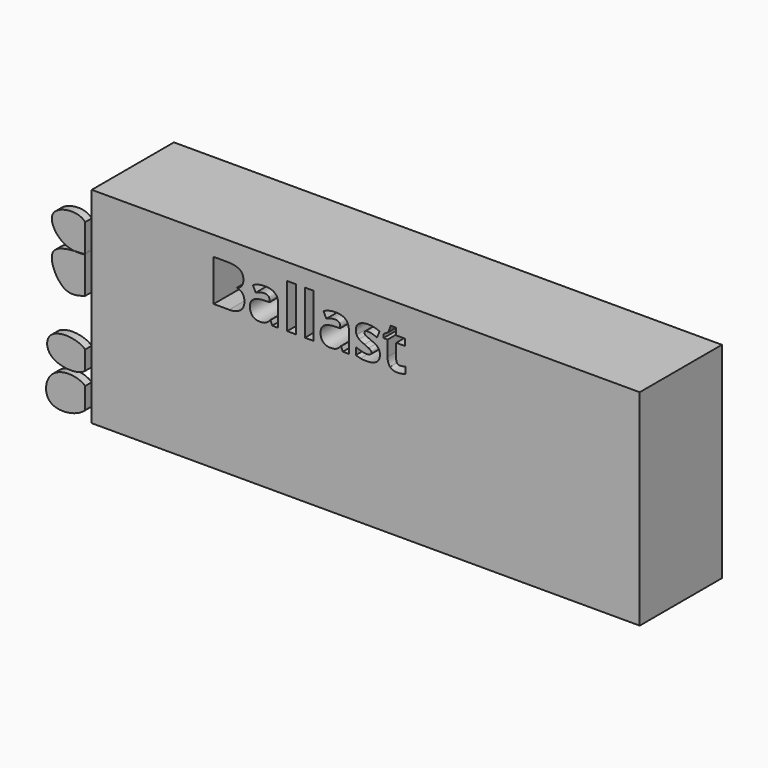
from build123d import *

# Parameters (mm, degrees)
F0_W     = 203.2
F0_H     = 76.2
F0_W_2   = 3.2102170287
F0_H_2   = 16.3812019001
F1_DEPTH = 38.1
F3_DEPTH = 3.048


with BuildPart() as f1:
    # F0 (on Front) → F1 (new body)
    with BuildSketch(Plane.XZ):
        with Locations((28.6630115066, 24.7132102959)):
            Rectangle(F0_W, F0_H)
        with BuildLine():
            Line((-27.7260044329, 40.2354274743), (-27.7260044329, 55.6262791053))
            Line((-27.7260044329, 55.6262791053), (-22.9359429272, 55.6262791053))
            add(Edge.make_bspline(
                [(-22.9359429272, 55.6262791053), (-19.6617236702, 55.6262791053), (-18.1829353432, 54.694878257)],
                knots=[0, 0, 0, 1, 1, 1], degree=2))
            add(Edge.make_bspline(
                [(-18.1829353432, 54.694878257), (-16.7041470162, 53.7634774087), (-16.7041470162, 51.7322487956)],
                knots=[0, 0, 0, 1, 1, 1], degree=2))
            add(Edge.make_bspline(
                [(-16.7041470162, 51.7322487956), (-16.7041470162, 50.3511480801), (-17.3509063756, 49.4669067684)],
                knots=[0, 0, 0, 1, 1, 1], degree=2))
            add(Edge.make_bspline(
                [(-17.3509063756, 49.4669067684), (-17.9976657351, 48.5826654567), (-19.0722294624, 48.4041329252)],
                knots=[0, 0, 0, 1, 1, 1], degree=2))
            Line((-19.0722294624, 48.4041329252), (-19.0722294624, 48.299708237))
            add(Edge.make_bspline(
                [(-19.0722294624, 48.299708237), (-17.6102838271, 47.972960019), (-16.9618401985, 47.0786130923)],
                knots=[0, 0, 0, 1, 1, 1], degree=2))
            add(Edge.make_bspline(
                [(-16.9618401985, 47.0786130923), (-16.3133965699, 46.1842661656), (-16.3133965699, 44.6987407619)],
                knots=[0, 0, 0, 1, 1, 1], degree=2))
            add(Edge.make_bspline(
                [(-16.3133965699, 44.6987407619), (-16.3133965699, 42.5934043055), (-17.8359758952, 41.4144158899)],
                knots=[0, 0, 0, 1, 1, 1], degree=2))
            add(Edge.make_bspline(
                [(-17.8359758952, 41.4144158899), (-19.3585552205, 40.2354274743), (-21.9691724264, 40.2354274743)],
                knots=[0, 0, 0, 1, 1, 1], degree=2))
            Line((-21.9691724264, 40.2354274743), (-27.7260044329, 40.2354274743))
        make_face(mode=Mode.SUBTRACT)
        with BuildLine():
            Line((-3.779065443, 40.2354274743), (-6.0191434326, 40.2354274743))
            Line((-6.0191434326, 40.2354274743), (-6.6423230237, 41.8354831812))
            Line((-6.6423230237, 41.8354831812), (-6.726536482, 41.8354831812))
            add(Edge.make_bspline(
                [(-6.726536482, 41.8354831812), (-7.5349856812, 40.8148160671), (-8.3939629554, 40.4190128133)],
                knots=[0, 0, 0, 1, 1, 1], degree=2))
            add(Edge.make_bspline(
                [(-8.3939629554, 40.4190128133), (-9.2529402297, 40.0232095595), (-10.6306724067, 40.0232095595)],
                knots=[0, 0, 0, 1, 1, 1], degree=2))
            add(Edge.make_bspline(
                [(-10.6306724067, 40.0232095595), (-12.3250471869, 40.0232095595), (-13.2985547643, 40.9933485986)],
                knots=[0, 0, 0, 1, 1, 1], degree=2))
            add(Edge.make_bspline(
                [(-13.2985547643, 40.9933485986), (-14.2720623418, 41.9634876378), (-14.2720623418, 43.7521814911)],
                knots=[0, 0, 0, 1, 1, 1], degree=2))
            add(Edge.make_bspline(
                [(-14.2720623418, 43.7521814911), (-14.2720623418, 45.6250888028), (-12.9617009313, 46.514382922)],
                knots=[0, 0, 0, 1, 1, 1], degree=2))
            add(Edge.make_bspline(
                [(-12.9617009313, 46.514382922), (-11.6513395208, 47.4036770412), (-9.0104054699, 47.4979961144)],
                knots=[0, 0, 0, 1, 1, 1], degree=2))
            Line((-9.0104054699, 47.4979961144), (-6.9657027034, 47.5619983427))
            Line((-6.9657027034, 47.5619983427), (-6.9657027034, 48.0773847072))
            add(Edge.make_bspline(
                [(-6.9657027034, 48.0773847072), (-6.9657027034, 49.8660785606), (-8.7981875551, 49.8660785606)],
                knots=[0, 0, 0, 1, 1, 1], degree=2))
            add(Edge.make_bspline(
                [(-8.7981875551, 49.8660785606), (-10.2096051155, 49.8660785606), (-12.1161978104, 49.013838363)],
                knots=[0, 0, 0, 1, 1, 1], degree=2))
            Line((-12.1161978104, 49.013838363), (-13.1772873844, 51.1831770477))
            add(Edge.make_bspline(
                [(-13.1772873844, 51.1831770477), (-11.1460587713, 52.2476351601), (-8.6735516369, 52.2476351601)],
                knots=[0, 0, 0, 1, 1, 1], degree=2))
            add(Edge.make_bspline(
                [(-8.6735516369, 52.2476351601), (-6.3054691907, 52.2476351601), (-5.0422673168, 51.2151781619)],
                knots=[0, 0, 0, 1, 1, 1], degree=2))
            add(Edge.make_bspline(
                [(-5.0422673168, 51.2151781619), (-3.779065443, 50.1827211636), (-3.779065443, 48.0773847072)],
                knots=[0, 0, 0, 1, 1, 1], degree=2))
            Line((-3.779065443, 48.0773847072), (-3.779065443, 40.2354274743))
        make_face(mode=Mode.SUBTRACT)
        with Locations((1.1339477117, 48.4260284244)):
            Rectangle(F0_W_2, F0_H_2, mode=Mode.SUBTRACT)
        with Locations((7.7127030708, 48.4260284244)):
            Rectangle(F0_W_2, F0_H_2, mode=Mode.SUBTRACT)
        with BuildLine():
            Line((22.4012144599, 40.2354274743), (20.1611364703, 40.2354274743))
            Line((20.1611364703, 40.2354274743), (19.5379568792, 41.8354831812))
            Line((19.5379568792, 41.8354831812), (19.4537434209, 41.8354831812))
            add(Edge.make_bspline(
                [(19.4537434209, 41.8354831812), (18.6452942217, 40.8148160671), (17.7863169474, 40.4190128133)],
                knots=[0, 0, 0, 1, 1, 1], degree=2))
            add(Edge.make_bspline(
                [(17.7863169474, 40.4190128133), (16.9273396732, 40.0232095595), (15.5496074961, 40.0232095595)],
                knots=[0, 0, 0, 1, 1, 1], degree=2))
            add(Edge.make_bspline(
                [(15.5496074961, 40.0232095595), (13.855232716, 40.0232095595), (12.8817251386, 40.9933485986)],
                knots=[0, 0, 0, 1, 1, 1], degree=2))
            add(Edge.make_bspline(
                [(12.8817251386, 40.9933485986), (11.9082175611, 41.9634876378), (11.9082175611, 43.7521814911)],
                knots=[0, 0, 0, 1, 1, 1], degree=2))
            add(Edge.make_bspline(
                [(11.9082175611, 43.7521814911), (11.9082175611, 45.6250888028), (13.2185789716, 46.514382922)],
                knots=[0, 0, 0, 1, 1, 1], degree=2))
            add(Edge.make_bspline(
                [(13.2185789716, 46.514382922), (14.5289403821, 47.4036770412), (17.169874433, 47.4979961144)],
                knots=[0, 0, 0, 1, 1, 1], degree=2))
            Line((17.169874433, 47.4979961144), (19.2145771995, 47.5619983427))
            Line((19.2145771995, 47.5619983427), (19.2145771995, 48.0773847072))
            add(Edge.make_bspline(
                [(19.2145771995, 48.0773847072), (19.2145771995, 49.8660785606), (17.3820923478, 49.8660785606)],
                knots=[0, 0, 0, 1, 1, 1], degree=2))
            add(Edge.make_bspline(
                [(17.3820923478, 49.8660785606), (15.9706747874, 49.8660785606), (14.0640820925, 49.013838363)],
                knots=[0, 0, 0, 1, 1, 1], degree=2))
            Line((14.0640820925, 49.013838363), (13.0029925184, 51.1831770477))
            add(Edge.make_bspline(
                [(13.0029925184, 51.1831770477), (15.0342211316, 52.2476351601), (17.506728266, 52.2476351601)],
                knots=[0, 0, 0, 1, 1, 1], degree=2))
            add(Edge.make_bspline(
                [(17.506728266, 52.2476351601), (19.8748107122, 52.2476351601), (21.1380125861, 51.2151781619)],
                knots=[0, 0, 0, 1, 1, 1], degree=2))
            add(Edge.make_bspline(
                [(21.1380125861, 51.2151781619), (22.4012144599, 50.1827211636), (22.4012144599, 48.0773847072)],
                knots=[0, 0, 0, 1, 1, 1], degree=2))
            Line((22.4012144599, 48.0773847072), (22.4012144599, 40.2354274743))
        make_face(mode=Mode.SUBTRACT)
        with BuildLine():
            add(Edge.make_bspline(
                [(33.6150785614, 45.2360226256), (33.9216155494, 44.6044216887), (33.9216155494, 43.7319702612)],
                knots=[0, 0, 0, 1, 1, 1], degree=2))
            add(Edge.make_bspline(
                [(33.9216155494, 43.7319702612), (33.9216155494, 41.9196966395), (32.6634664831, 40.9714530995)],
                knots=[0, 0, 0, 1, 1, 1], degree=2))
            add(Edge.make_bspline(
                [(32.6634664831, 40.9714530995), (31.4053174167, 40.0232095595), (28.899124899, 40.0232095595)],
                knots=[0, 0, 0, 1, 1, 1], degree=2))
            add(Edge.make_bspline(
                [(28.899124899, 40.0232095595), (27.6157117952, 40.0232095595), (26.7095749843, 40.1983735527)],
                knots=[0, 0, 0, 1, 1, 1], degree=2))
            add(Edge.make_bspline(
                [(26.7095749843, 40.1983735527), (25.8034381735, 40.3735375459), (25.0152002042, 40.7103913789)],
                knots=[0, 0, 0, 1, 1, 1], degree=2))
            Line((25.0152002042, 40.7103913789), (25.0152002042, 43.3614310448))
            add(Edge.make_bspline(
                [(25.0152002042, 43.3614310448), (25.9078628617, 42.9403637535), (27.0295861257, 42.6557222646)],
                knots=[0, 0, 0, 1, 1, 1], degree=2))
            add(Edge.make_bspline(
                [(27.0295861257, 42.6557222646), (28.1513093897, 42.3710807757), (29.0035495872, 42.3710807757)],
                knots=[0, 0, 0, 1, 1, 1], degree=2))
            add(Edge.make_bspline(
                [(29.0035495872, 42.3710807757), (30.7518209807, 42.3710807757), (30.7518209807, 43.3816422748)],
                knots=[0, 0, 0, 1, 1, 1], degree=2))
            add(Edge.make_bspline(
                [(30.7518209807, 43.3816422748), (30.7518209807, 43.7622871061), (30.5193918359, 43.9997690584)],
                knots=[0, 0, 0, 1, 1, 1], degree=2))
            add(Edge.make_bspline(
                [(30.5193918359, 43.9997690584), (30.2869626911, 44.2372510107), (29.7193639824, 44.5370509221)],
                knots=[0, 0, 0, 1, 1, 1], degree=2))
            add(Edge.make_bspline(
                [(29.7193639824, 44.5370509221), (29.1517652738, 44.8368508335), (28.205206003, 45.2343383565)],
                knots=[0, 0, 0, 1, 1, 1], degree=2))
            add(Edge.make_bspline(
                [(28.205206003, 45.2343383565), (26.8476850559, 45.8036213343), (26.2093470423, 46.2886908538)],
                knots=[0, 0, 0, 1, 1, 1], degree=2))
            add(Edge.make_bspline(
                [(26.2093470423, 46.2886908538), (25.5710090287, 46.7737603734), (25.2829990015, 47.4003085028)],
                knots=[0, 0, 0, 1, 1, 1], degree=2))
            add(Edge.make_bspline(
                [(25.2829990015, 47.4003085028), (24.9949889742, 48.0268566323), (24.9949889742, 48.9397305198)],
                knots=[0, 0, 0, 1, 1, 1], degree=2))
            add(Edge.make_bspline(
                [(24.9949889742, 48.9397305198), (24.9949889742, 50.5094693817), (26.2093470423, 51.3667623867)],
                knots=[0, 0, 0, 1, 1, 1], degree=2))
            add(Edge.make_bspline(
                [(26.2093470423, 51.3667623867), (27.4237051103, 52.2240553918), (29.6570460233, 52.2240553918)],
                knots=[0, 0, 0, 1, 1, 1], degree=2))
            add(Edge.make_bspline(
                [(29.6570460233, 52.2240553918), (31.7825937097, 52.2240553918), (33.7936110929, 51.2977073509)],
                knots=[0, 0, 0, 1, 1, 1], degree=2))
            Line((33.7936110929, 51.2977073509), (32.8268405921, 48.9835215181))
            add(Edge.make_bspline(
                [(32.8268405921, 48.9835215181), (31.9409150112, 49.360797811), (31.1728882719, 49.6033325708)],
                knots=[0, 0, 0, 1, 1, 1], degree=2))
            add(Edge.make_bspline(
                [(31.1728882719, 49.6033325708), (30.4048615326, 49.8458673306), (29.60314941, 49.8458673306)],
                knots=[0, 0, 0, 1, 1, 1], degree=2))
            add(Edge.make_bspline(
                [(29.60314941, 49.8458673306), (28.1816262347, 49.8458673306), (28.1816262347, 49.0778405913)],
                knots=[0, 0, 0, 1, 1, 1], degree=2))
            add(Edge.make_bspline(
                [(28.1816262347, 49.0778405913), (28.1816262347, 48.646667685), (28.6397474476, 48.330025082)],
                knots=[0, 0, 0, 1, 1, 1], degree=2))
            add(Edge.make_bspline(
                [(28.6397474476, 48.330025082), (29.0978686605, 48.0133824789), (30.6473962924, 47.3935714262)],
                knots=[0, 0, 0, 1, 1, 1], degree=2))
            add(Edge.make_bspline(
                [(30.6473962924, 47.3935714262), (32.0251284695, 46.8343940633), (32.6668350214, 46.3510088129)],
                knots=[0, 0, 0, 1, 1, 1], degree=2))
            add(Edge.make_bspline(
                [(32.6668350214, 46.3510088129), (33.3085415733, 45.8676235625), (33.6150785614, 45.2360226256)],
                knots=[0, 0, 0, 1, 1, 1], degree=2))
        make_face(mode=Mode.SUBTRACT)
        with BuildLine():
            add(Edge.make_bspline(
                [(40.3656293752, 42.9100469086), (40.7496427449, 42.5832986905), (41.382927951, 42.5832986905)],
                knots=[0, 0, 0, 1, 1, 1], degree=2))
            add(Edge.make_bspline(
                [(41.382927951, 42.5832986905), (42.2250625336, 42.5832986905), (43.4040509492, 42.9504693685)],
                knots=[0, 0, 0, 1, 1, 1], degree=2))
            Line((43.4040509492, 42.9504693685), (43.4040509492, 40.5621756924))
            add(Edge.make_bspline(
                [(43.4040509492, 40.5621756924), (42.2048513036, 40.0232095595), (40.4565799102, 40.0232095595)],
                knots=[0, 0, 0, 1, 1, 1], degree=2))
            add(Edge.make_bspline(
                [(40.4565799102, 40.0232095595), (38.5297759852, 40.0232095595), (37.650587481, 40.9984014061)],
                knots=[0, 0, 0, 1, 1, 1], degree=2))
            add(Edge.make_bspline(
                [(37.650587481, 40.9984014061), (36.7713989768, 41.9735932528), (36.7713989768, 43.9206084077)],
                knots=[0, 0, 0, 1, 1, 1], degree=2))
            Line((36.7713989768, 43.9206084077), (36.7713989768, 49.5932269558))
            Line((36.7713989768, 49.5932269558), (35.2353454982, 49.5932269558))
            Line((35.2353454982, 49.5932269558), (35.2353454982, 50.9507479029))
            Line((35.2353454982, 50.9507479029), (37.0038281216, 52.0253116303))
            Line((37.0038281216, 52.0253116303), (37.9301761625, 54.511292918))
            Line((37.9301761625, 54.511292918), (39.9816160056, 54.511292918))
            Line((39.9816160056, 54.511292918), (39.9816160056, 52.0051004003))
            Line((39.9816160056, 52.0051004003), (43.2760464926, 52.0051004003))
            Line((43.2760464926, 52.0051004003), (43.2760464926, 49.5932269558))
            Line((43.2760464926, 49.5932269558), (39.9816160056, 49.5932269558))
            Line((39.9816160056, 49.5932269558), (39.9816160056, 43.9206084077))
            add(Edge.make_bspline(
                [(39.9816160056, 43.9206084077), (39.9816160056, 43.2367951266), (40.3656293752, 42.9100469086)],
                knots=[0, 0, 0, 1, 1, 1], degree=2))
        make_face(mode=Mode.SUBTRACT)
    extrude(amount=F1_DEPTH)


with BuildPart() as f3:
    # F2 (on face) → F3 (new body)
    with BuildSketch(Plane.XZ.offset(38.1)):
        with BuildLine():
            add(Edge.make_bspline(
                [(-72.9369884934, 42.9982505739), (-72.9369884934, 38.464145114), (-72.9369884934, 33.9300396542), (-72.9369884934, 29.3959341943)],
                knots=[0.3886371851, 0.3886371851, 0.3886371851, 0.3886371851, 13.9909535646, 13.9909535646, 13.9909535646, 13.9909535646], degree=3))
            add(Edge.make_bspline(
                [(-76.963987331, 42.787935422), (-74.9299485972, 42.5262813223), (-73.2010111806, 42.7910800658), (-72.9369884934, 42.9982505739)],
                knots=[0.5748651015, 0.5748651015, 0.5748651015, 0.5748651015, 0.7099314681, 0.7099314681, 0.7099314681, 0.7099314681], degree=3))
            add(Edge.make_bspline(
                [(-76.963987331, 42.787935422), (-80.835579424, 42.4894615948), (-88.2006509729, 40.9207531865), (-81.5055520215, 26.8162053465), (-75.6275506776, 28.5858893297), (-72.9369884934, 29.3959341943)],
                knots=[0.0922489301, 0.0922489301, 0.0922489301, 0.0922489301, 0.3674266003, 0.7104495273, 1, 1, 1, 1], degree=3))
        make_face()
    extrude(amount=F3_DEPTH)


with BuildPart() as f3b:
    # F2 (on face) → F3, piece 2 (new body)
    with BuildSketch(Plane.XZ.offset(38.1)):
        with BuildLine():
            add(Edge.make_bspline(
                [(-72.9369884934, 42.9982505739), (-74.3015431268, 42.9431222958), (-75.6660977602, 42.8879940176), (-76.963987331, 42.787935422)],
                knots=[0, 0, 0, 0, 0.0922489301, 0.0922489301, 0.0922489301, 0.0922489301], degree=3))
            add(Edge.make_bspline(
                [(-72.9369884934, 43.386887759), (-72.9369884934, 43.2573420306), (-72.9369884934, 43.1277963022), (-72.9369884934, 42.9982505739)],
                knots=[0, 0, 0, 0, 0.3886371851, 0.3886371851, 0.3886371851, 0.3886371851], degree=3))
            add(Edge.make_bspline(
                [(-72.9369884934, 43.386887759), (-72.9372100552, 43.3997580293), (-72.9372078172, 43.4131166204), (-72.9369884934, 43.426955209)],
                knots=[0.757491309, 0.757491309, 0.757491309, 0.757491309, 0.7599408785, 0.7599408785, 0.7599408785, 0.7599408785], degree=3))
            Line((-72.9369884934, 43.426955209), (-72.9369884934, 53.4914657474))
            add(Edge.make_bspline(
                [(-72.9369884934, 53.4914657474), (-75.2530333111, 56.47610757), (-89.3241990524, 54.8744083699), (-83.1774574412, 44.2022407672), (-78.0699322925, 42.9302016574), (-76.963987331, 42.787935422)],
                knots=[0, 0, 0, 0, 0.261284451, 0.5014269879, 0.5748651015, 0.5748651015, 0.5748651015, 0.5748651015], degree=3))
        make_face()
    extrude(amount=F3_DEPTH)


with BuildPart() as f3c:
    # F2 (on face) → F3, piece 3 (new body)
    with BuildSketch(Plane.XZ.offset(38.1)):
        with BuildLine():
            Line((-72.9369884934, 4.9117649905), (-72.9369884934, 11.9072422385))
            add(Edge.make_bspline(
                [(-72.9369884934, 11.9072422385), (-75.8148304456, 14.5820180066), (-87.5706896239, 15.314116017), (-87.5706896165, 3.3275242949), (-75.8148304462, 2.5954255371), (-72.9369884934, 4.9117649905)],
                knots=[0, 0, 0, 0, 0.2860532775, 0.4999999963, 0.7860532741, 0.7860532741, 0.7860532741, 0.7860532741], degree=3))
        make_face()
    extrude(amount=F3_DEPTH)


with BuildPart() as f3d:
    # F2 (on face) → F3, piece 4 (new body)
    with BuildSketch(Plane.XZ.offset(38.1)):
        with BuildLine():
            Line((-72.9369884934, -7.9132756218), (-72.9369884934, 0))
            add(Edge.make_bspline(
                [(-72.9369884934, 0), (-75.7335327511, 2.520720827), (-87.3034007051, 2.9967160526), (-88.8498976312, -12.9398829385), (-75.9330143958, -10.9219102957), (-72.9369884934, -7.9132756218)],
                knots=[0, 0, 0, 0, 0.2680499522, 0.5056296372, 0.7831631995, 0.7831631995, 0.7831631995, 0.7831631995], degree=3))
        make_face()
    extrude(amount=F3_DEPTH)


solid = Compound([f1.part, f3.part, f3b.part, f3c.part, f3d.part])
